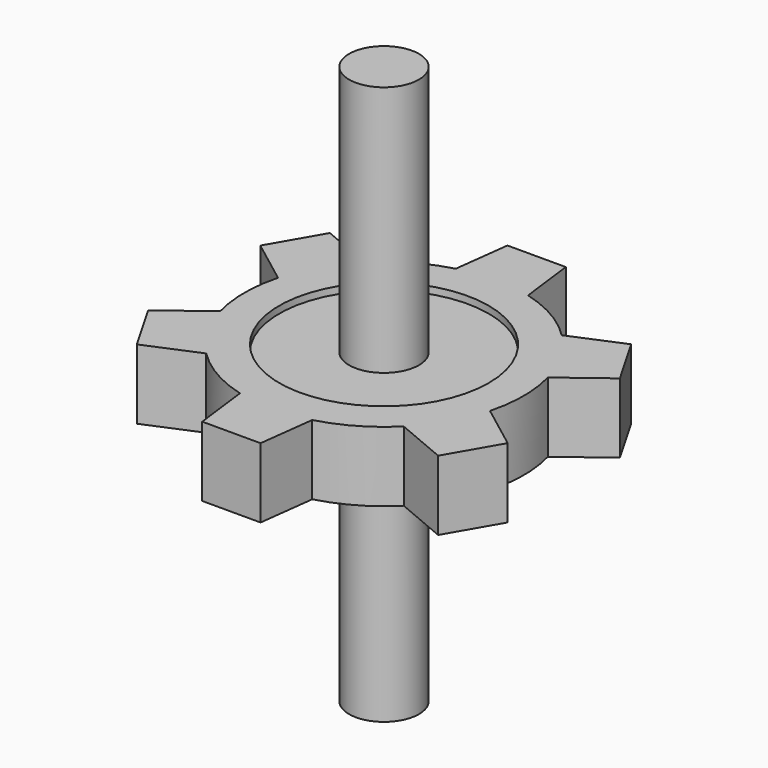
from build123d import *

# Parameters (mm, degrees)
F0_R       = 25.4
F1_DEPTH   = 6.35
F3_DEPTH   = 12.7
F4_SIZE2   = 1.26999
F4_SIZE    = 10.15999
F4_2_SIZE2 = 1.26999
F4_2_SIZE  = 10.15999
F6_COUNT   = 6
F7_R       = 19.05
F7_R_2     = 6.35
F8_DEPTH   = 1.27
F9_DEPTH   = 25.4
F10_R      = 6.35
F11_DEPTH  = 50.8


# Not quite as in the source:
# - a fillet or chamfer is up to 0.001 mm smaller than in the source, because OpenCascade refuses the exact size
# - a pattern or mirror of a feature is missing from the dataset's text; its kind, count and spacing are read off the source's solid


with BuildPart() as f1:
    # F0 (on Top) → F1 (new body, symmetric)
    with BuildSketch(Plane.XY):
        Circle(F0_R)
    extrude(amount=F1_DEPTH, both=True)

    # F2 (on face) → F3 (join)
    with BuildSketch(Plane.XY.offset(6.35)):
        with BuildLine():
            ThreePointArc((-6.5740037456, 24.5345159877), (0, 25.4), (6.5740037456, 24.5345159877))
            Line((6.5740037456, 24.5345159877), (6.5740037456, 34.6945159877))
            Line((6.5740037456, 34.6945159877), (-6.5740037456, 34.6945159877))
            Line((-6.5740037456, 34.6945159877), (-6.5740037456, 24.5345159877))
        make_face()
    extrude(amount=-F3_DEPTH)

    # F4 (size 10.16 and 1.27 in the source; OpenCascade refuses exactly that, so slightly less here)
    f4_edges = [f1.edges().sort_by_distance(p)[0] for p in [
        (6.574004, 34.694516, 0),
    ]]
    f4_side = f1.faces().sort_by_distance((6.574004, 29.614516, 0))[0]
    chamfer(f4_edges, length=F4_SIZE, length2=F4_SIZE2, reference=f4_side)

    # F4#2 (size 10.16 and 1.27 in the source; OpenCascade refuses exactly that, so slightly less here)
    f4_2_edges = [f1.edges().sort_by_distance(p)[0] for p in [
        (-6.574004, 34.694516, 0),
    ]]
    f4_2_side = f1.faces().sort_by_distance((-6.574004, 29.614516, 0))[0]
    chamfer(f4_2_edges, length=F4_2_SIZE, length2=F4_2_SIZE2, reference=f4_2_side)

    # F6: F1 ×6 about axis
    f6_axis = Axis((0, 0, 22.000901401), (0, 0, 1))


with BuildPart() as f1_1:
    add(f1.part)
    for i in range(1, F6_COUNT):
        add(f1.part.rotate(f6_axis, i * 360 / F6_COUNT))

    # F7 (on face) → F8 (cut)
    with BuildSketch(Plane.XY.offset(6.35)):
        Circle(F7_R)
        Circle(F7_R_2, mode=Mode.SUBTRACT)
        Circle(F7_R_2)
    f8 = extrude(amount=-F8_DEPTH, mode=Mode.SUBTRACT)

    # F8_copies: F8 across plane
    add(f8.mirror(Plane(origin=(0, 0, 0), x_dir=(-1, 0, 0), z_dir=(0, 0, -1))), mode=Mode.SUBTRACT)

    # F7 (on face) → F9 (cut)
    with BuildSketch(Plane.XY.offset(6.35)):
        Circle(F7_R_2)
    extrude(amount=-F9_DEPTH, mode=Mode.SUBTRACT)


with BuildPart() as f11:
    # F10 (on Top) → F11 (new body, symmetric)
    with BuildSketch(Plane.XY):
        Circle(F10_R)
    extrude(amount=F11_DEPTH, both=True)


solid = Compound([f1_1.part, f11.part])
